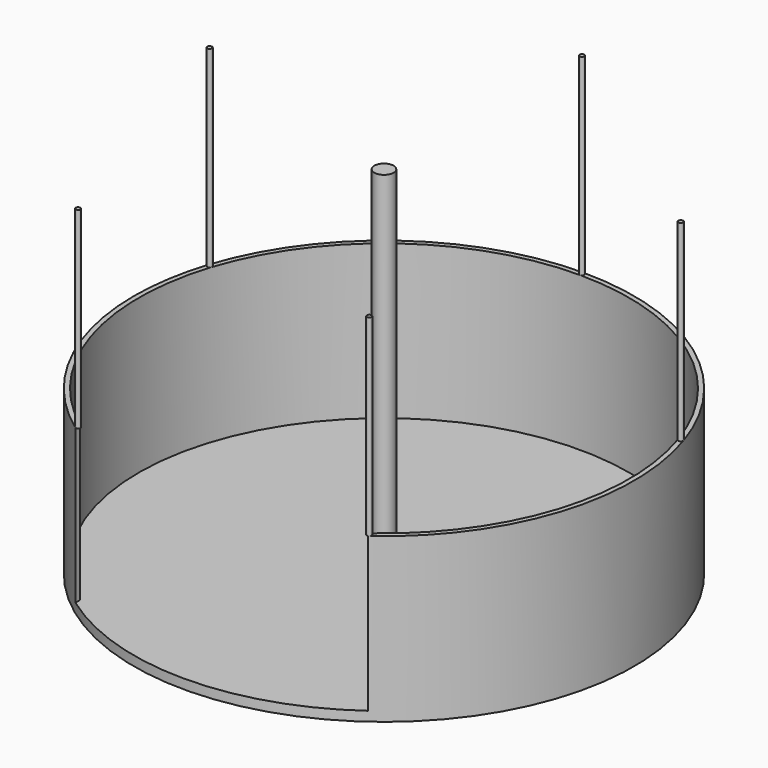
from build123d import *

# Parameters (mm, degrees)
F4_DEPTH        = 101.6027760721
F5_R            = 1.5875
F6_DEPTH        = 127
F6_COPIES_COUNT = 5


# Not quite as in the source:
# - a pattern or mirror of a feature is missing from the dataset's text; its kind, count and spacing are read off the source's solid


with BuildPart() as f2:
    # F1 (on Front) → F2 (revolve)
    with BuildSketch(Plane.XZ):
        Polygon((-161.925, 101.2154587421), (-165.1, 101.2154587421), (-165.1, -0.3845412579), (-165.1, -6.7345412579), (0, -6.7345412579), (0, 0), (0, 228.6), (-6.35, 228.6), (-6.35, -0.3873173299), (-161.925, -0.3873173299), align=None)
    revolve(axis=Axis((0, 0, 5.5167637765), (0, 0, -1)))

    # F3 (on face) → F4 (cut, through all)
    with BuildSketch(Plane.XY.offset(101.2154587421)):
        with BuildLine():
            ThreePointArc((96.6025192728, -129.9525255435), (0, -161.925), (-96.6025192728, -129.9525255435))
            Line((-96.6025192728, -129.9525255435), (-96.6025192728, -133.8878757399))
            ThreePointArc((-96.6025192728, -133.8878757399), (0, -165.1), (96.6025192728, -133.8878757399))
            Line((96.6025192728, -133.8878757399), (96.6025192728, -129.9525255435))
        make_face()
    extrude(amount=-F4_DEPTH, mode=Mode.SUBTRACT)

    # F5 (on face) → F6 (join)
    with BuildSketch(Plane.XY.offset(101.2154587421)):
        with Locations((0, 163.5125)):
            Circle(F5_R)
    f6 = extrude(amount=F6_DEPTH)

    # F6_copies: F6 ×5 about axis
    f6_copies_axis = Axis((0, 0, 0), (0, 0, 1))
    for i in range(1, F6_COPIES_COUNT):
        add(f6.rotate(f6_copies_axis, i * 360 / F6_COPIES_COUNT))


solid = f2.part
